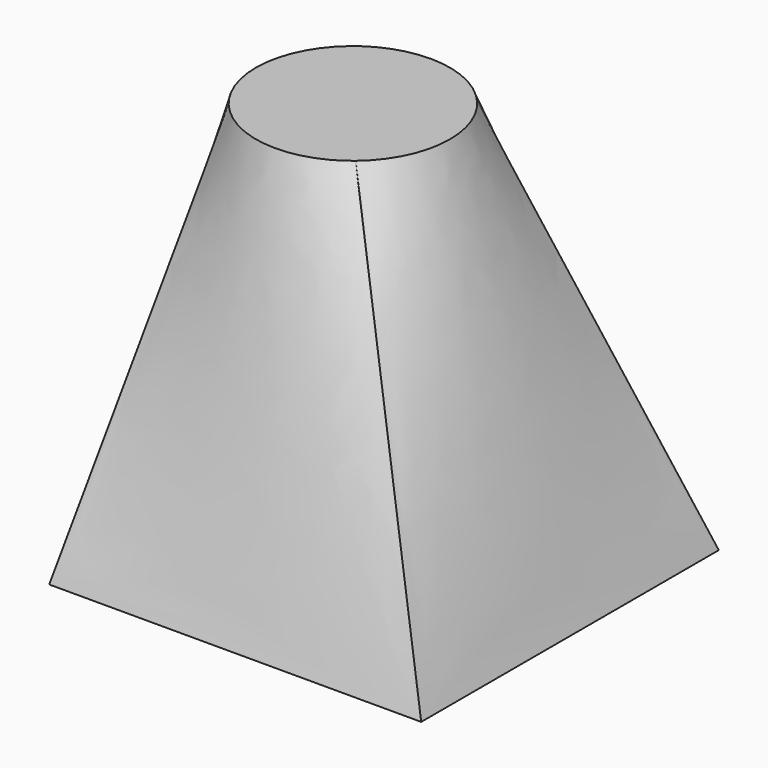
from build123d import *

# Parameters (mm, degrees)
F0_W = 111.4384680986
F0_H = 111.4384680986


# Not quite as in the source:
# - the arcs of a loft's sections are written as splines that run evenly, so that the points pair up as in the source's solid


with BuildPart() as f3:
    # F0 (on Top) → F3 section 0
    with BuildSketch(Plane.XY):
        with Locations((6.6977106035, 9.633474052)):
            Rectangle(F0_W, F0_H)
    # F2 (on offset) → F3 section 1
    with BuildSketch(Plane.XY.offset(115.824)):
        with BuildLine():
            add(Edge.make_bspline(
                [(-25.4332735487, 37.1479816271), (-26.8926824867, 35.9274449641), (-28.2318459417, 34.563202801), (-30.6183497695, 31.599600895), (-31.6656311314, 30.000314433), (-33.4281089071, 26.6280735063), (-34.1432617404, 24.855202427), (-35.2139824316, 21.2039158074), (-35.5695238139, 19.3255905523), (-35.9073402249, 15.5355751367), (-35.8896069004, 13.6239786919), (-35.4815369359, 9.8408826475), (-35.0912103863, 7.9694765923), (-33.9529359462, 4.3386821784), (-33.2050162019, 2.5793835981), (-31.3802805346, -0.7595797922), (-30.3035097318, -2.3391620399), (-29.0829730688, -3.7985709779)],
                knots=[0, 0, 0, 0, 0.125, 0.125, 0.25, 0.25, 0.375, 0.375, 0.5, 0.5, 0.625, 0.625, 0.75, 0.75, 0.875, 0.875, 1, 1, 1, 1], degree=3))
            add(Edge.make_bspline(
                [(-29.0829730688, -3.7985709779), (-27.8624364057, -5.257979916), (-26.4981942427, -6.597143371), (-23.5345923367, -8.9836471988), (-21.9353058746, -10.0309285606), (-18.563064948, -11.7934063364), (-16.7901938687, -12.5085591696), (-13.1389072491, -13.5792798609), (-11.2605819939, -13.9348212432), (-7.4705665784, -14.2726376542), (-5.5589701336, -14.2549043297), (-1.7758740892, -13.8468343652), (0.095531966, -13.4565078155), (3.72632638, -12.3182333755), (5.4856249602, -11.5703136311), (8.8245883506, -9.7455779638), (10.4041705982, -8.6688071611), (11.8635795362, -7.448270498)],
                knots=[0, 0, 0, 0, 0.125, 0.125, 0.25, 0.25, 0.375, 0.375, 0.5, 0.5, 0.625, 0.625, 0.75, 0.75, 0.875, 0.875, 1, 1, 1, 1], degree=3))
            add(Edge.make_bspline(
                [(11.8635795362, -7.448270498), (13.3229884743, -6.227733835), (14.6621519293, -4.863491672), (17.0486557571, -1.899889766), (18.095937119, -0.3006033039), (19.8584148947, 3.0716376228), (20.573567728, 4.844508702), (21.6442884192, 8.4957953217), (21.9998298015, 10.3741205768), (22.3376462125, 14.1641359923), (22.319912888, 16.0757324371), (21.9118429235, 19.8588284816), (21.5215163739, 21.7302345367), (20.3832419338, 25.3610289507), (19.6353221895, 27.120327531), (17.8105865222, 30.4592909213), (16.7338157194, 32.0388731689), (15.5132790564, 33.498282107)],
                knots=[0, 0, 0, 0, 0.125, 0.125, 0.25, 0.25, 0.375, 0.375, 0.5, 0.5, 0.625, 0.625, 0.75, 0.75, 0.875, 0.875, 1, 1, 1, 1], degree=3))
            add(Edge.make_bspline(
                [(15.5132790564, 33.498282107), (14.2927423933, 34.957691045), (12.9285002303, 36.2968545), (9.9648983243, 38.6833583279), (8.3656118622, 39.7306396897), (4.9933709356, 41.4931174655), (3.2204998563, 42.2082702987), (-0.4307867633, 43.2789909899), (-2.3091120185, 43.6345323723), (-6.099127434, 43.9723487833), (-8.0107238788, 43.9546154587), (-11.7938199232, 43.5465454943), (-13.6652259784, 43.1562189446), (-17.2960203924, 42.0179445045), (-19.0553189726, 41.2700247602), (-22.394282363, 39.4452890929), (-23.9738646106, 38.3685182902), (-25.4332735487, 37.1479816271)],
                knots=[0, 0, 0, 0, 0.125, 0.125, 0.25, 0.25, 0.375, 0.375, 0.5, 0.5, 0.625, 0.625, 0.75, 0.75, 0.875, 0.875, 1, 1, 1, 1], degree=3))
        make_face()
    loft(ruled=True)


solid = f3.part
